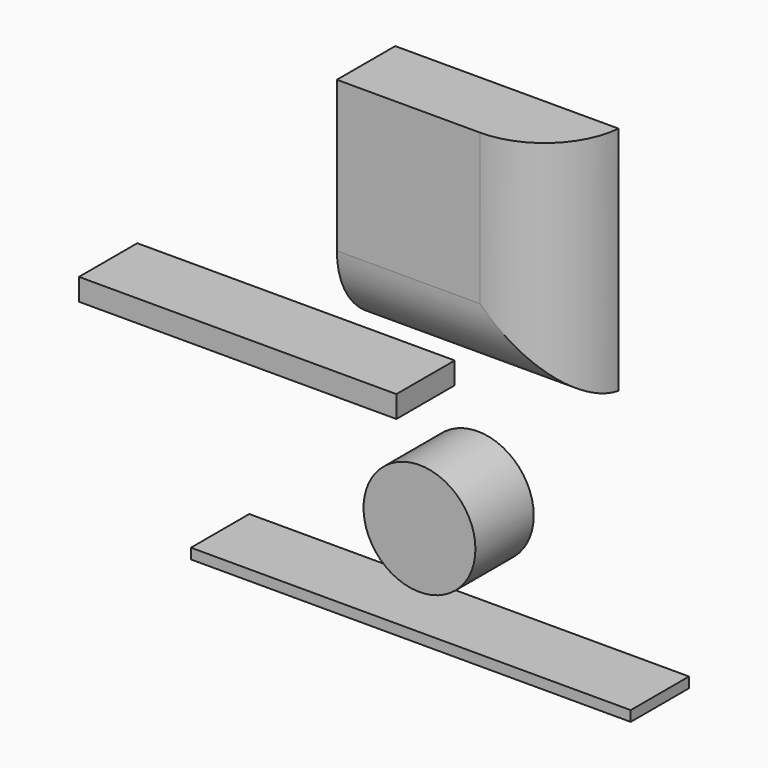
from build123d import *

# Parameters (mm, degrees)
F0_W        = 110.8502186835
F0_H        = 2.6185084134
F1_DEPTH    = 18.3726
F0_W_2      = 56.3120255373
F0_H_2      = 58.1890968606
F0_R        = 14.0994798806
F2_T1_DEPTH = 157.4443686872
F3_T1_DEPTH = 139.0949713805


# Not quite as in the source:
# - a fillet or chamfer that OpenCascade refuses, or shapes differently, is made with other operations: its cross-section is extruded or revolved along the edge and cut away or added


with BuildPart() as f1:
    # F0 (on Front) → F1 (new body)
    with BuildSketch(Plane.XZ):
        with Locations((14.9836894125, -51.6428193077)):
            Rectangle(F0_W, F0_H)
    extrude(amount=F1_DEPTH)


with BuildPart() as f1b:
    # F0 (on Front) → F1, piece 2 (new body)
    with BuildSketch(Plane.XZ):
        with Locations((24.5051165048, 36.3681823947)):
            Rectangle(F0_W_2, F0_H_2)
    extrude(amount=F1_DEPTH)

    # F2: fillet of radius 20.32 on 1 edges, made by hand

    # F2_s2 → F2_t1 (cut)
    with BuildSketch(Plane.YZ.offset(-54.2170678388)):
        with BuildLine():
            ThreePointArc((0, 7.2736339644), (-13.0937696354, 13.8375400236), (-18.3726, 27.5001025944))
            Line((-18.3726, 27.5001025944), (-18.3726, 7.2736339644))
            Line((-18.3726, 7.2736339644), (0, 7.2736339644))
        make_face()
    extrude(amount=F2_T1_DEPTH, mode=Mode.SUBTRACT)

    # F3: fillet of radius 20.32 on 1 edges, made by hand

    # F3_s2 → F3_t1 (cut)
    with BuildSketch(Plane.XY.offset(-23.0660689806)):
        with BuildLine():
            ThreePointArc((52.6611292735, 0), (46.0972232142, -13.0937696354), (32.4346606435, -18.3726))
            Line((32.4346606435, -18.3726), (52.6611292735, -18.3726))
            Line((52.6611292735, -18.3726), (52.6611292735, 0))
        make_face()
    extrude(amount=F3_T1_DEPTH, mode=Mode.SUBTRACT)


with BuildPart() as f1c:
    # F0 (on Front) → F1, piece 3 (new body)
    with BuildSketch(Plane.XZ):
        with Locations((17.1657819301, -27.3488722742)):
            Circle(F0_R)
    extrude(amount=F1_DEPTH)


with BuildPart() as f1d:
    # F0 (on Front) → F1, piece 4 (new body)
    with BuildSketch(Plane.XZ):
        Polygon((-68.6631277204, -4.9460716546), (11.3468747586, -4.9460716546), (11.3468747586, 0), (11.3468747586, 0.5818922073), (-68.6631277204, 0.5818922073), align=None)
    extrude(amount=F1_DEPTH)


solid = Compound([f1.part, f1b.part, f1c.part, f1d.part])
